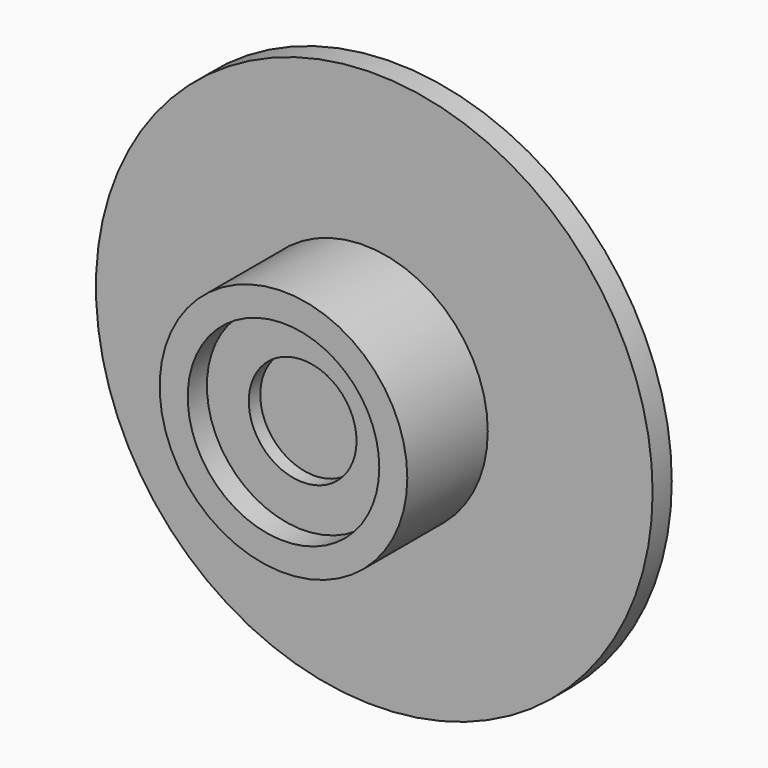
from build123d import *

# Parameters (mm, degrees)
F0_R      = 51.7
F0_R_2    = 40
F0_R_3    = 22.5
F1_DEPTH  = 57
F2_DEPTH  = 10
F3_DEPTH  = 16
F4_R      = 50
F4_R_2    = 45
F5_DEPTH  = 37
F6_DEPTH  = 41
F4_R_3    = 100
F4_R_4    = 92
F4_R_5    = 60
F4_R_6    = 51.7
F7_DEPTH  = 5
F8_DEPTH  = 3
F9_R      = 116.2259856664
F10_DEPTH = 10


# Not quite as in the source:
# - a feature names something its author has since deleted; it is built from what else it names


with BuildPart() as f1:
    # F0 (on Front) → F1 (new body)
    with BuildSketch(Plane.XZ):
        Circle(F0_R)
        Circle(F0_R_2, mode=Mode.SUBTRACT)
        Circle(F0_R_2)
        Circle(F0_R_3, mode=Mode.SUBTRACT)
        Circle(F0_R_3)
    extrude(amount=-F1_DEPTH)

    # F0 (on Front) → F2 (cut)
    with BuildSketch(Plane.XZ):
        Circle(F0_R_2)
        Circle(F0_R_3, mode=Mode.SUBTRACT)
    extrude(amount=-F2_DEPTH, mode=Mode.SUBTRACT)

    # F0 (on Front) → F3 (cut)
    with BuildSketch(Plane.XZ):
        Circle(F0_R_3)
    extrude(amount=-F3_DEPTH, mode=Mode.SUBTRACT)

    # F4 (on face) → F5 (cut)
    with BuildSketch(Plane(origin=(0, 57, 0), x_dir=(-1, 0, 0), z_dir=(0, 1, 0))):
        Circle(F4_R)
        Circle(F4_R_2, mode=Mode.SUBTRACT)
    extrude(amount=-F5_DEPTH, mode=Mode.SUBTRACT)

    # F4 (on face) → F6 (cut)
    with BuildSketch(Plane(origin=(0, 57, 0), x_dir=(-1, 0, 0), z_dir=(0, 1, 0))):
        Circle(F4_R_2)
    extrude(amount=-F6_DEPTH, mode=Mode.SUBTRACT)

    # F4 (on face) → F7 (join)
    with BuildSketch(Plane(origin=(0, 57, 0), x_dir=(-1, 0, 0), z_dir=(0, 1, 0))):
        Circle(F4_R_3)
        Circle(F4_R_4, mode=Mode.SUBTRACT)
        Circle(F4_R_4)
        Circle(F4_R_5, mode=Mode.SUBTRACT)
        Circle(F4_R_5)
        Circle(F4_R_6, mode=Mode.SUBTRACT)
    extrude(amount=-F7_DEPTH)

    # F4 (on face) → F8 (cut)
    with BuildSketch(Plane(origin=(0, 57, 0), x_dir=(-1, 0, 0), z_dir=(0, 1, 0))):
        Circle(F4_R_4)
        Circle(F4_R_5, mode=Mode.SUBTRACT)
    extrude(amount=-F8_DEPTH, mode=Mode.SUBTRACT)

    # F9 (on face) → F10 (join)
    with BuildSketch(Plane.XZ.offset(-52)):
        with Locations((4.3108635582, 0)):
            Circle(F9_R)
    extrude(amount=F10_DEPTH)


solid = f1.part
